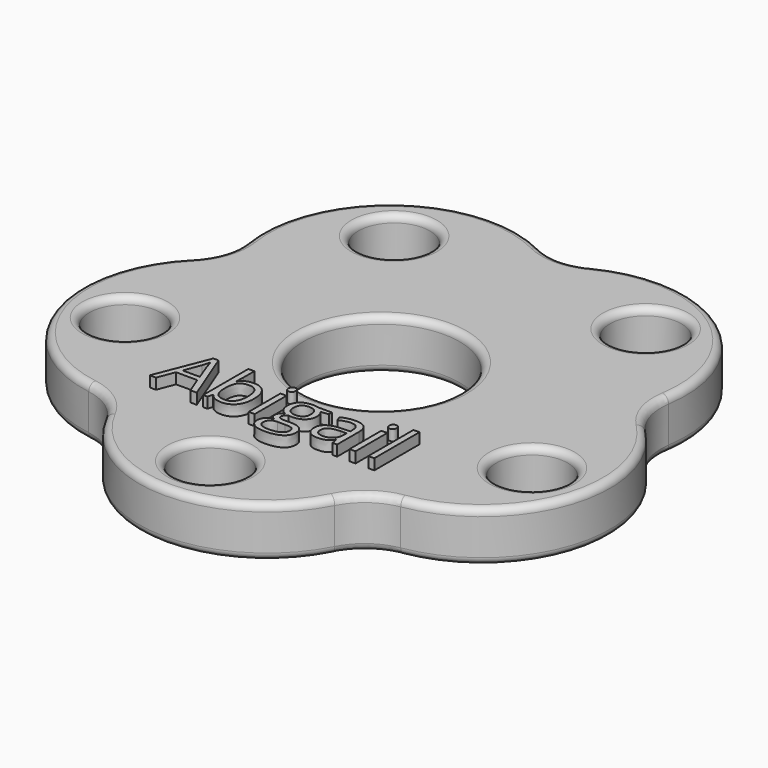
from build123d import *

# Parameters (mm, degrees)
F0_R         = 5
F0_R_2       = 10.95
F1_DEPTH     = 7.05
F2_R         = 8
F3_R         = 1
F4_TEXT_SIZE = 10.4166666667
F5_DEPTH     = 1.5
F6_TEXT_SIZE = 6.9444444444
F7_DEPTH     = 0.5


# Not quite as in the source:
# - Text() gives the source's letters only with a copy of the font that has no kerning and outlines rounded to 1/6400 em; it was checked with that copy


with BuildPart() as f1:
    # F0 (on Top) → F1 (new body)
    with BuildSketch(Plane.XY):
        with BuildLine():
            ThreePointArc((28.3522424721, 9.2122020116), (22.3358395871, 30.7426457862), (0, 29.8113119319))
            ThreePointArc((0, 29.8113119319), (-22.3358395871, 30.7426457862), (-28.3522424721, 9.2122020116))
            ThreePointArc((-28.3522424721, 9.2122020116), (-36.1401476192, -11.7426457862), (-17.5226495051, -24.1178579775))
            ThreePointArc((-17.5226495051, -24.1178579775), (0, -38), (17.5226495051, -24.1178579775))
            ThreePointArc((17.5226495051, -24.1178579775), (36.1401476192, -11.7426457862), (28.3522424721, 9.2122020116))
        make_face()
        with Locations((-28.5316954889, -9.2705098312)):
            Circle(F0_R, mode=Mode.SUBTRACT)
        with Locations((0, -30)):
            Circle(F0_R, mode=Mode.SUBTRACT)
        with Locations((28.5316954889, -9.2705098313)):
            Circle(F0_R, mode=Mode.SUBTRACT)
        with Locations((-17.6335575688, 24.2705098312)):
            Circle(F0_R, mode=Mode.SUBTRACT)
        Circle(F0_R_2, mode=Mode.SUBTRACT)
        with Locations((17.6335575688, 24.2705098312)):
            Circle(F0_R, mode=Mode.SUBTRACT)
    extrude(amount=F1_DEPTH)

    # F2
    f2_edges = [f1.edges().sort_by_distance(p)[0] for p in [
        (17.52265, -24.117858, 3.525),
        (28.352242, 9.212202, 3.525),
        (0, 29.811312, 3.525),
        (-28.352242, 9.212202, 3.525),
        (-17.52265, -24.117858, 3.525),
    ]]
    fillet(f2_edges, radius=F2_R)

    # F3
    f3_edges = [f1.edges().sort_by_distance(p)[0] for p in [
        (0, -38, 7.05),
        (-18.439369, -25.379614, 7.05),
        (18.439369, -25.379614, 7.05),
        (-36.140148, -11.742646, 7.05),
        (36.140148, -11.742646, 7.05),
        (-29.835526, 9.69415, 7.05),
        (29.835526, 9.69415, 7.05),
        (-22.33584, 30.742646, 7.05),
        (22.33584, 30.742646, 7.05),
        (0, 31.370928, 7.05),
        (-33.531695, -9.27051, 7.05),
        (-5, -30, 7.05),
        (23.531695, -9.27051, 7.05),
        (-22.633558, 24.27051, 7.05),
        (-10.95, 0, 7.05),
        (12.633558, 24.27051, 7.05),
        (0, -38, 0),
        (-18.439369, -25.379614, 0),
        (18.439369, -25.379614, 0),
        (-36.140148, -11.742646, 0),
        (36.140148, -11.742646, 0),
        (-29.835526, 9.69415, 0),
        (29.835526, 9.69415, 0),
        (-22.33584, 30.742646, 0),
        (22.33584, 30.742646, 0),
        (0, 31.370928, 0),
        (-33.531695, -9.27051, 0),
        (-5, -30, 0),
        (23.531695, -9.27051, 0),
        (-22.633558, 24.27051, 0),
        (-10.95, 0, 0),
        (12.633558, 24.27051, 0),
    ]]
    fillet(f3_edges, radius=F3_R)

    # F4 (on face) → F5 (join)
    with BuildSketch(Plane.XY.offset(7.05)):
        with Locations((-16.0799153646, -20.5)):
            Text('Abigail', F4_TEXT_SIZE, font='Open Sans', text_align=(TextAlign.LEFT, TextAlign.BOTTOM))
    extrude(amount=F5_DEPTH)

    # F6 (on face) → F7 (cut)
    with BuildSketch(Plane(origin=(0, 0, 0), x_dir=(1, 0, 0), z_dir=(0, 0, -1))):
        with Locations((-29.8311414931, -6.2623811968)):
            Text('Jesus              Loves', F6_TEXT_SIZE, font='Open Sans', text_align=(TextAlign.LEFT, TextAlign.BOTTOM))
        with Locations((-7.0643446181, -29.7959150001)):
            Text('You!', F6_TEXT_SIZE, font='Open Sans', text_align=(TextAlign.LEFT, TextAlign.BOTTOM))
    extrude(amount=-F7_DEPTH, mode=Mode.SUBTRACT)


solid = f1.part
